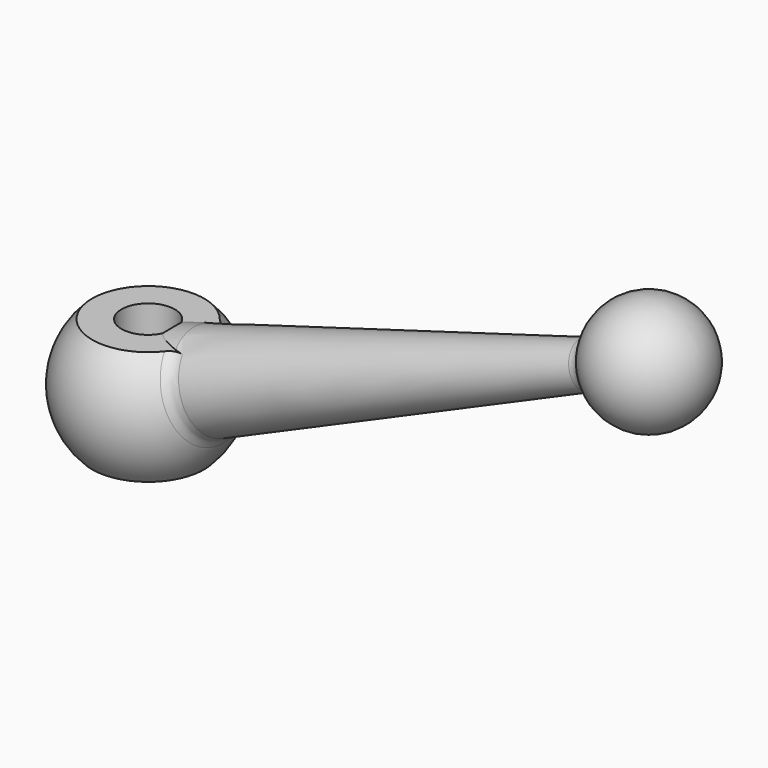
from build123d import *

# Parameters (mm, degrees)
F3_T4_ANGLE = 342.0779351193
F5_D        = 14


# Not quite as in the source:
# - a fillet or chamfer that OpenCascade refuses, or shapes differently, is made with other operations: its cross-section is extruded or revolved along the edge and cut away or added


with BuildPart() as f1:
    # F0 (on Front) → F1 (revolve)
    with BuildSketch(Plane.XZ):
        with BuildLine():
            Line((0, 15), (-14.6969384567, 15))
            ThreePointArc((-14.6969384567, 15), (-21, 0), (-14.6969384567, -15))
            Line((-14.6969384567, -15), (0, -15))
            Line((0, -15), (0, -14.1738577821))
            Line((0, -14.1738577821), (0, 0))
            Line((0, 0), (0, 13.5706276966))
            Line((0, 13.5706276966), (0, 15))
        make_face()
    revolve(axis=Axis((0, 0, 0), (0, 0, -1)))

    # F0 (on Front) → F2 (revolve)
    with BuildSketch(Plane.XZ):
        with BuildLine():
            Line((116.5621770938, 48.278140652), (12.0901276659, 17.1705798686))
            Line((12.0901276659, 17.1705798686), (4.800423118, 15))
            Line((4.800423118, 15), (0, 13.5706276966))
            Line((0, 13.5706276966), (0, 0))
            Line((0, 0), (19.7335450365, 7.1824230098))
            Line((19.7335450365, 7.1824230098), (117.4615775982, 42.7525179157))
            ThreePointArc((117.4615775982, 42.7525179157), (116.7518070973, 45.4729978899), (116.5621770938, 48.278140652))
        make_face()
        with BuildLine():
            ThreePointArc((145.6523562218, 53.0131222155), (129.1471447343, 62.6879798784), (116.5621770938, 48.278140652))
            ThreePointArc((116.5621770938, 48.278140652), (116.7518070973, 45.4729978899), (117.4615775982, 42.7525179157))
            Line((117.4615775982, 42.7525179157), (145.6523562218, 53.0131222155))
        make_face()
    revolve(axis=Axis((72.8261781109, 0, 26.5065611077), (0.9396926208, 0, 0.3420201433)))

    # F3: fillet of radius 5 on 2 edges, made by hand


with BuildPart() as f3_tool2:
    # F3_s3 → F3_t4 (revolve)
    with BuildSketch(Plane(origin=(1e-10, -2.3e-09, -3e-10), x_dir=(-0.9985488213, -0.053853982, 0), z_dir=(-0.0532739776, 0.9877945051, 0.1463690505))):
        with BuildLine():
            ThreePointArc((-10.2959142188, 18.3028453824), (-12.2007985149, 17.6906243055), (-14.1932009283, 17.8742855481))
            Line((-14.1932009283, 17.8742855481), (-12.0219430441, 17.2183880011))
            ThreePointArc((-12.0219430441, 17.2183880011), (-11.1720947014, 17.7815718865), (-10.2959142188, 18.3028453824))
        make_face()
    revolve(axis=Axis((16.194369394, 1.4e-09, 5.8942683966), (0.9396926208, 0, 0.3420201433)), revolution_arc=F3_T4_ANGLE)

    split(bisect_by=Plane.XY.offset(15), keep=Keep.BOTTOM)


with BuildPart() as f1_1:
    add(f1.part)

    # F3_t1: union F3_tool2
    add(f3_tool2.part)

    # F3_s6 → F3_t7 (revolve)
    with BuildSketch(Plane.XZ):
        with BuildLine():
            ThreePointArc((113.4424776902, 47.3492200522), (115.6809078185, 48.7404946697), (116.9009348123, 51.0766771615))
            ThreePointArc((116.9009348123, 51.0766771615), (116.6656687231, 49.6853844353), (116.5621770938, 48.278140652))
            Line((116.5621770938, 48.278140652), (113.4424776902, 47.3492200522))
        make_face()
    revolve(axis=Axis((118.4432878821, 0, 43.1098312377), (0.9396926208, 0, 0.3420201433)))

    # F5 (through all)
    with Locations(Plane(origin=(0, 0, -15), x_dir=(1, 0, 0), z_dir=(0, 0, -1))):
        with Locations((0, 0)):
            Hole(F5_D / 2)


solid = f1_1.part
